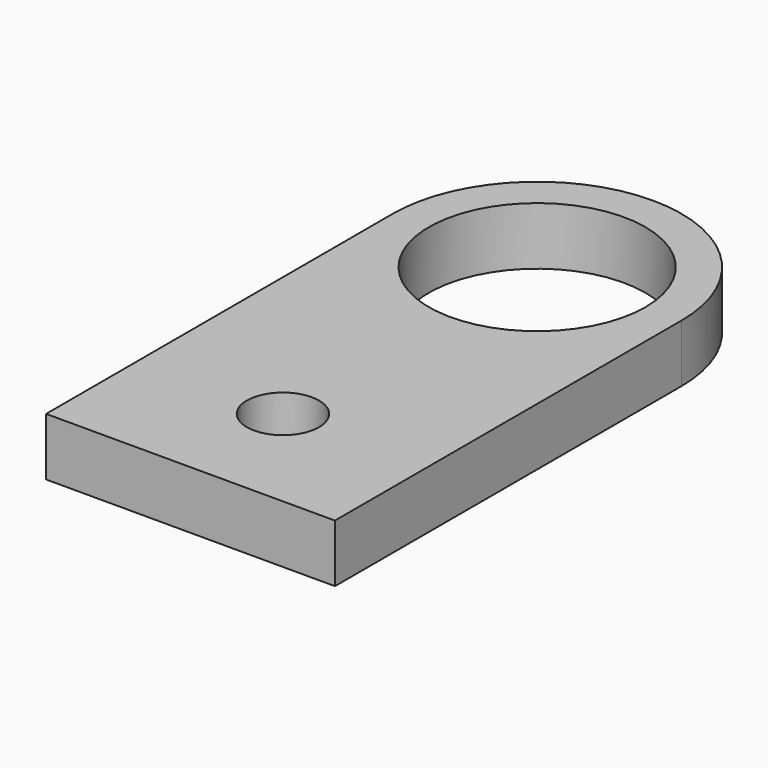
from build123d import *

# Parameters (mm, degrees)
F0_W     = 20
F0_H     = 40
F0_R     = 2.5
F0_R_2   = 7.5
F1_DEPTH = 4
F2_R     = 9.99999


# Not quite as in the source:
# - a fillet or chamfer is up to 0.001 mm smaller than in the source, because OpenCascade refuses the exact size


with BuildPart() as f1:
    # F0 (on Top) → F1 (new body)
    with BuildSketch(Plane.XY):
        with Locations((10, 20)):
            Rectangle(F0_W, F0_H)
        with Locations((10, 8)):
            Circle(F0_R, mode=Mode.SUBTRACT)
        with Locations((10, 30)):
            Circle(F0_R_2, mode=Mode.SUBTRACT)
    extrude(amount=F1_DEPTH)

    # F2 (radius 10 in the source; OpenCascade refuses exactly that, so slightly less here)
    f2_edges = [f1.edges().sort_by_distance(p)[0] for p in [
        (20, 40, 2),
        (0, 40, 2),
    ]]
    fillet(f2_edges, radius=F2_R)


solid = f1.part
